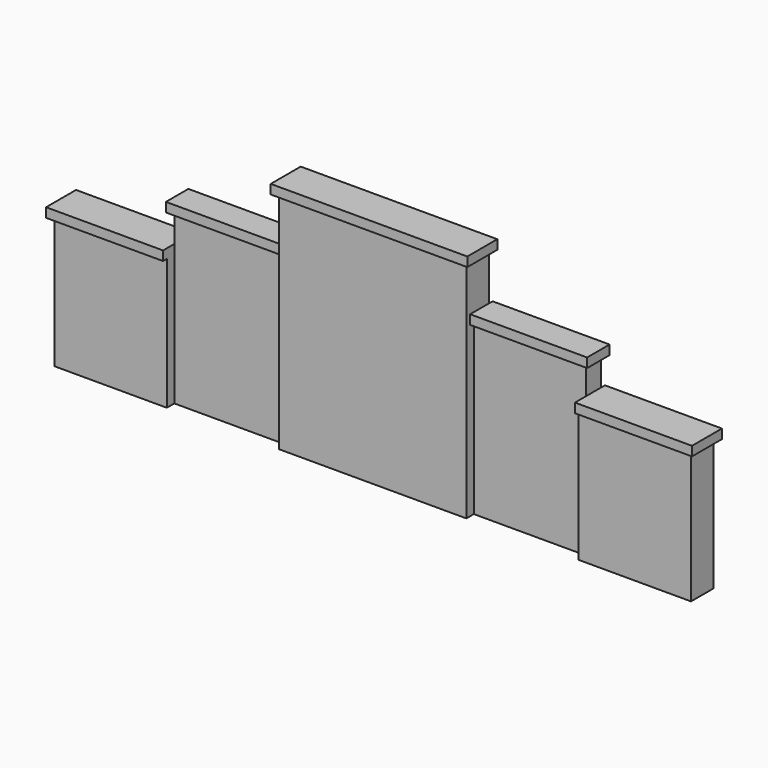
from build123d import *

# Parameters (mm, degrees)
F0_W     = 76.2
F0_H     = 88.9
F1_DEPTH = 19.05
F0_H_2   = 25.4
F2_DEPTH = 12.7
F0_W_2   = 127
F0_H_3   = 38.1
F3_DEPTH = 19.05
F4_W     = 79.375
F4_H     = 25.4
F5_DEPTH = 6.35
F6_W     = 76.2
F6_H     = 12.7
F6_W_2   = 79.375
F6_H_2   = 19.05
F7_DEPTH = 6.35
F8_W     = 133.35
F8_H     = 25.4
F8_W_2   = 127
F8_H_2   = 19.05
F9_DEPTH = 6.35


with BuildPart() as f1:
    # F0 (on Front) → F1 (new body)
    with BuildSketch(Plane.XZ):
        with Locations((-177.8, 44.45)):
            Rectangle(F0_W, F0_H)
    extrude(amount=F1_DEPTH)

    # F0 (on Front) → F2 (join)
    with BuildSketch(Plane.XZ):
        with Locations((-101.6, 44.45)):
            Rectangle(F0_W, F0_H)
        with Locations((-101.6, 101.6)):
            Rectangle(F0_W, F0_H_2)
    extrude(amount=F2_DEPTH)



with BuildPart() as f1b:
    # F0 (on Front) → F1, piece 2 (new body)
    with BuildSketch(Plane.XZ):
        with Locations((177.8, 44.45)):
            Rectangle(F0_W, F0_H)
    extrude(amount=F1_DEPTH)

    # F0 (on Front) → F2, piece 2 (join)
    with BuildSketch(Plane.XZ):
        with Locations((101.6, 101.6)):
            Rectangle(F0_W, F0_H_2)
        with Locations((101.6, 44.45)):
            Rectangle(F0_W, F0_H)
    extrude(amount=F2_DEPTH)


with BuildPart() as f1_1:
    add(f1.part)

    add(f1b.part)  # F3 merges F1b
    # F0 (on Front) → F3 (join)
    with BuildSketch(Plane.XZ):
        with Locations((0, 133.35)):
            Rectangle(F0_W_2, F0_H_3)
        with Locations((0, 101.6)):
            Rectangle(F0_W_2, F0_H_2)
        with Locations((0, 44.45)):
            Rectangle(F0_W_2, F0_H)
    extrude(amount=F3_DEPTH)

    # F4 (on face) → F5 (join)
    with BuildSketch(Plane.XY.offset(88.9)):
        Polygon((-139.7, 3.175), (-219.075, 3.175), (-219.075, -22.225), (-139.7, -22.225), (-139.7, -19.05), (-215.9, -19.05), (-215.9, 0), (-139.7, 0), align=None)
        Polygon((-139.7, -12.7), (-139.7, 0), (-215.9, 0), (-215.9, -19.05), (-139.7, -19.05), align=None)
        with Locations((179.3875, -9.525)):
            Rectangle(F4_W, F4_H)
    extrude(amount=F5_DEPTH)

    # F6 (on face) → F7 (join)
    with BuildSketch(Plane.XY.offset(114.3)):
        Polygon((-63.5, 3.175), (-142.875, 3.175), (-142.875, -15.875), (-63.5, -15.875), (-63.5, -12.7), (-139.7, -12.7), (-139.7, 0), (-63.5, 0), align=None)
        with Locations((-101.6, -6.35)):
            Rectangle(F6_W, F6_H)
        with Locations((103.1875, -6.35)):
            Rectangle(F6_W_2, F6_H_2)
    extrude(amount=F7_DEPTH)

    # F8 (on face) → F9 (join)
    with BuildSketch(Plane.XY.offset(152.4)):
        with Locations((0, -9.525)):
            Rectangle(F8_W, F8_H)
        with Locations((0, -9.525)):
            Rectangle(F8_W_2, F8_H_2, mode=Mode.SUBTRACT)
        with Locations((0, -9.525)):
            Rectangle(F8_W_2, F8_H_2)
    extrude(amount=F9_DEPTH)


solid = f1_1.part
